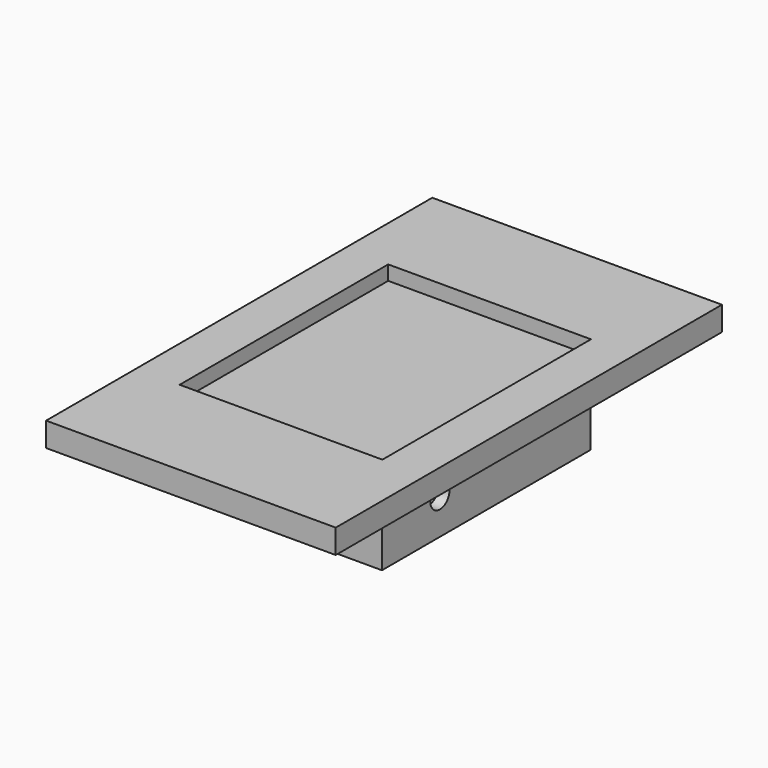
from build123d import *

# Parameters (mm, degrees)
F1_DEPTH = 19.05
F2_W     = 47.8625434434
F2_H     = 13.97
F3_DEPTH = 60.96
F4_DEPTH = 6.35
F6_D     = 6.35
F8_DEPTH = 3.81


# Not quite as in the source:
# - a feature names something its author has since deleted; it is built from what else it names


with BuildPart() as f1:
    # F0 (on Top) → F1 (new body)
    with BuildSketch(Plane.XY):
        Polygon((-0.0274520135, 33.8990125982), (-26.4712717217, 33.8990125982), (-26.4712717217, -0.3909874018), (-26.4712717217, -34.6809874018), (16.3237974048, -34.6809874018), (26.8687282783, -34.6809874018), (26.8687282783, -0.3909874018), (26.8687282783, 33.8990125982), align=None)
    extrude(amount=-F1_DEPTH)

    # F2 (on face) → F3 (cut)
    with BuildSketch(Plane(origin=(0, 33.8990125982, 0), x_dir=(-1, 0, 0), z_dir=(0, 1, 0))):
        with Locations((0, -9.525)):
            Rectangle(F2_W, F2_H)
    extrude(amount=-F3_DEPTH, mode=Mode.SUBTRACT)

    # F0 (on Top) → F4 (join)
    with BuildSketch(Plane.XY):
        Polygon((-26.4712717217, -0.3909874018), (-26.4712717217, 33.8990125982), (-0.0274520135, 33.8990125982), (-0.0274520135, 37.7090125982), (-0.0274520135, 63.1090125982), (-38.1274520135, 63.1090125982), (-38.1274520135, -63.8909874018), (16.3237974048, -63.8909874018), (16.3237974048, -34.6809874018), (-26.4712717217, -34.6809874018), align=None)
        Polygon((-0.0274520135, 33.8990125982), (-26.4712717217, 33.8990125982), (-26.4712717217, -0.3909874018), (-26.4712717217, -34.6809874018), (16.3237974048, -34.6809874018), (26.8687282783, -34.6809874018), (26.8687282783, -0.3909874018), (26.8687282783, 33.8990125982), align=None)
        Polygon((-0.0274520135, 37.7090125982), (-0.0274520135, 33.8990125982), (26.8687282783, 33.8990125982), (26.8687282783, -0.3909874018), (38.0725479865, -0.3909874018), (38.0725479865, 63.1090125982), (-0.0274520135, 63.1090125982), align=None)
        Polygon((38.0725479865, -0.3909874018), (26.8687282783, -0.3909874018), (26.8687282783, -34.6809874018), (16.3237974048, -34.6809874018), (16.3237974048, -63.8909874018), (38.0725479865, -63.8909874018), align=None)
    extrude(amount=F4_DEPTH)

    # F6 (through all)
    with Locations(Plane.YZ.offset(26.8687282783)):
        with Locations((-15.6309874018, -9.525)):
            Hole(F6_D / 2)

    # F7 (on face) → F8 (cut)
    with BuildSketch(Plane.XY.offset(6.35)):
        Polygon((26.67, -34.29), (26.67, 0), (26.67, 34.29), (-26.67, 34.29), (-26.67, 0), (-26.67, -34.29), align=None)
    extrude(amount=-F8_DEPTH, mode=Mode.SUBTRACT)


solid = f1.part
